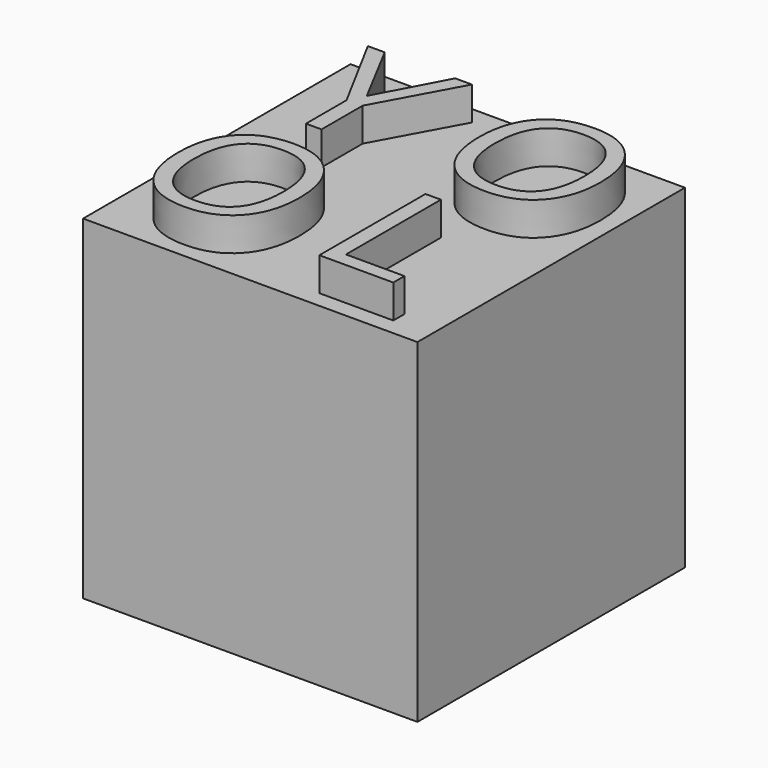
from build123d import *

# Parameters (mm, degrees)
F0_W         = 25.4
F0_H         = 25.4
F1_DEPTH     = 25.4
F2_TEXT_SIZE = 14.1111111111
F3_DEPTH     = 2.54


# Not quite as in the source:
# - Text() gives the source's letters only with a copy of the font that has no kerning and outlines rounded to 1/6400 em; it was checked with that copy


with BuildPart() as f1:
    # F0 (on Top) → F1 (new body)
    with BuildSketch(Plane.XY):
        Rectangle(F0_W, F0_H)
    extrude(amount=F1_DEPTH)

    # F2 (on face) → F3 (join)
    with BuildSketch(Plane.XY.offset(25.4)):
        with Locations((-10.3011111111, 1.27)):
            Text('Y', F2_TEXT_SIZE, font='Open Sans', text_align=(TextAlign.LEFT, TextAlign.BOTTOM))
        with Locations((1.2854340278, 1.27)):
            Text('O', F2_TEXT_SIZE, font='Open Sans', text_align=(TextAlign.LEFT, TextAlign.BOTTOM))
        with Locations((2.8497829861, -11.43)):
            Text('L', F2_TEXT_SIZE, font='Open Sans', text_align=(TextAlign.LEFT, TextAlign.BOTTOM))
        with Locations((-11.4145659722, -11.43)):
            Text('O', F2_TEXT_SIZE, font='Open Sans', text_align=(TextAlign.LEFT, TextAlign.BOTTOM))
    extrude(amount=F3_DEPTH)


solid = f1.part
